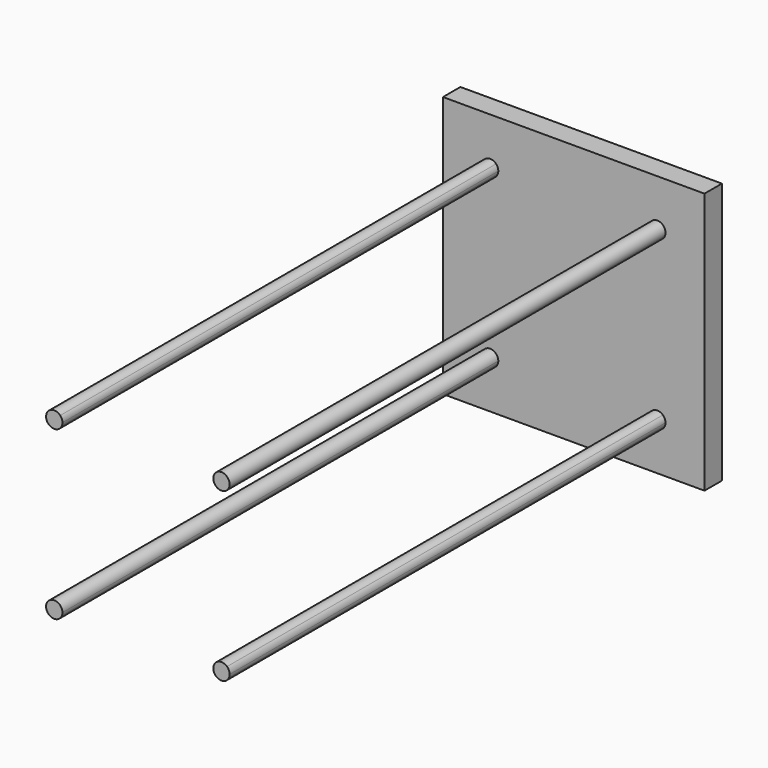
from build123d import *

# Parameters (mm, degrees)
F0_W     = 304.8
F0_H     = 304.8
F1_DEPTH = 25.4
F2_DEPTH = 660.4


with BuildPart() as f1:
    # F0 (on Front) → F1 (new body)
    with BuildSketch(Plane.XZ):
        with Locations((-11.4630328134, -11.4630328134)):
            Rectangle(F0_W, F0_H)
        with BuildLine():
            ThreePointArc((92.4711311021, 79.0087948248), (117.5894180385, 36.8373497331), (126.3319671866, -11.4630328134))
            ThreePointArc((126.3319671866, -11.4630328134), (117.5894180385, -59.7634153598), (92.4711311021, -101.9348604515))
            ThreePointArc((92.4711311021, -101.9348604515), (94.708384089, -105.1022008793), (95.4977461002, -108.898811727))
            ThreePointArc((95.4977461002, -108.898811727), (89.4651656842, -117.7604498627), (79.0087948248, -115.3971967289))
            ThreePointArc((79.0087948248, -115.3971967289), (-11.4630328134, -149.2580328134), (-101.9348604515, -115.3971967289))
            ThreePointArc((-101.9348604515, -115.3971967289), (-115.6340038178, -115.6340038178), (-115.3971967289, -101.9348604515))
            ThreePointArc((-115.3971967289, -101.9348604515), (-149.2580328134, -11.4630328134), (-115.3971967289, 79.0087948248))
            ThreePointArc((-115.3971967289, 79.0087948248), (-115.6340038178, 92.707938191), (-101.9348604515, 92.4711311021))
            ThreePointArc((-101.9348604515, 92.4711311021), (-11.4630328134, 126.3319671866), (79.0087948248, 92.4711311021))
            ThreePointArc((79.0087948248, 92.4711311021), (89.4651656842, 94.834384236), (95.4977461002, 85.9727461002))
            ThreePointArc((95.4977461002, 85.9727461002), (94.708384089, 82.1761352526), (92.4711311021, 79.0087948248))
        make_face(mode=Mode.SUBTRACT)
        with BuildLine():
            ThreePointArc((92.4711311021, -101.9348604515), (117.5894180385, -59.7634153598), (126.3319671866, -11.4630328134))
            ThreePointArc((126.3319671866, -11.4630328134), (117.5894180385, 36.8373497331), (92.4711311021, 79.0087948248))
            ThreePointArc((92.4711311021, 79.0087948248), (79.2375540094, 79.2375540094), (79.0087948248, 92.4711311021))
            ThreePointArc((79.0087948248, 92.4711311021), (-11.4630328134, 126.3319671866), (-101.9348604515, 92.4711311021))
            ThreePointArc((-101.9348604515, 92.4711311021), (-100.0371735912, 89.4651656842), (-99.373811727, 85.9727461002))
            ThreePointArc((-99.373811727, 85.9727461002), (-105.1022008793, 77.2371081114), (-115.3971967289, 79.0087948248))
            ThreePointArc((-115.3971967289, 79.0087948248), (-149.2580328134, -11.4630328134), (-115.3971967289, -101.9348604515))
            ThreePointArc((-115.3971967289, -101.9348604515), (-105.1022008793, -100.1631737382), (-99.373811727, -108.898811727))
            ThreePointArc((-99.373811727, -108.898811727), (-100.0371735912, -112.391231311), (-101.9348604515, -115.3971967289))
            ThreePointArc((-101.9348604515, -115.3971967289), (-11.4630328134, -149.2580328134), (79.0087948248, -115.3971967289))
            ThreePointArc((79.0087948248, -115.3971967289), (79.2375540094, -102.1636196362), (92.4711311021, -101.9348604515))
        make_face()
        with BuildLine():
            ThreePointArc((79.0087948248, 92.4711311021), (79.2375540094, 79.2375540094), (92.4711311021, 79.0087948248))
            ThreePointArc((92.4711311021, 79.0087948248), (85.9727461002, 85.9727461002), (79.0087948248, 92.4711311021))
        make_face()
    extrude(amount=F1_DEPTH)

    # F0 (on Front) → F2 (join)
    with BuildSketch(Plane.XZ):
        with BuildLine():
            ThreePointArc((79.0087948248, 92.4711311021), (79.2375540094, 79.2375540094), (92.4711311021, 79.0087948248))
            ThreePointArc((92.4711311021, 79.0087948248), (85.9727461002, 85.9727461002), (79.0087948248, 92.4711311021))
        make_face()
        with BuildLine():
            ThreePointArc((79.0087948248, 92.4711311021), (85.9727461002, 85.9727461002), (92.4711311021, 79.0087948248))
            ThreePointArc((92.4711311021, 79.0087948248), (94.708384089, 82.1761352526), (95.4977461002, 85.9727461002))
            ThreePointArc((95.4977461002, 85.9727461002), (89.4651656842, 94.834384236), (79.0087948248, 92.4711311021))
        make_face()
        with BuildLine():
            ThreePointArc((95.4977461002, -108.898811727), (94.708384089, -105.1022008793), (92.4711311021, -101.9348604515))
            ThreePointArc((92.4711311021, -101.9348604515), (85.9727461002, -108.898811727), (79.0087948248, -115.3971967289))
            ThreePointArc((79.0087948248, -115.3971967289), (89.4651656842, -117.7604498627), (95.4977461002, -108.898811727))
        make_face()
        with BuildLine():
            ThreePointArc((79.0087948248, -115.3971967289), (85.9727461002, -108.898811727), (92.4711311021, -101.9348604515))
            ThreePointArc((92.4711311021, -101.9348604515), (79.2375540094, -102.1636196362), (79.0087948248, -115.3971967289))
        make_face()
        with BuildLine():
            ThreePointArc((-99.373811727, 85.9727461002), (-100.0371735912, 89.4651656842), (-101.9348604515, 92.4711311021))
            ThreePointArc((-101.9348604515, 92.4711311021), (-108.898811727, 85.9727461002), (-115.3971967289, 79.0087948248))
            ThreePointArc((-115.3971967289, 79.0087948248), (-105.1022008793, 77.2371081114), (-99.373811727, 85.9727461002))
        make_face()
        with BuildLine():
            ThreePointArc((-115.3971967289, 79.0087948248), (-108.898811727, 85.9727461002), (-101.9348604515, 92.4711311021))
            ThreePointArc((-101.9348604515, 92.4711311021), (-115.6340038178, 92.707938191), (-115.3971967289, 79.0087948248))
        make_face()
        with BuildLine():
            ThreePointArc((-115.3971967289, -101.9348604515), (-115.6340038178, -115.6340038178), (-101.9348604515, -115.3971967289))
            ThreePointArc((-101.9348604515, -115.3971967289), (-108.898811727, -108.898811727), (-115.3971967289, -101.9348604515))
        make_face()
        with BuildLine():
            ThreePointArc((-115.3971967289, -101.9348604515), (-108.898811727, -108.898811727), (-101.9348604515, -115.3971967289))
            ThreePointArc((-101.9348604515, -115.3971967289), (-100.0371735912, -112.391231311), (-99.373811727, -108.898811727))
            ThreePointArc((-99.373811727, -108.898811727), (-105.1022008793, -100.1631737382), (-115.3971967289, -101.9348604515))
        make_face()
    extrude(amount=F2_DEPTH)


solid = f1.part
